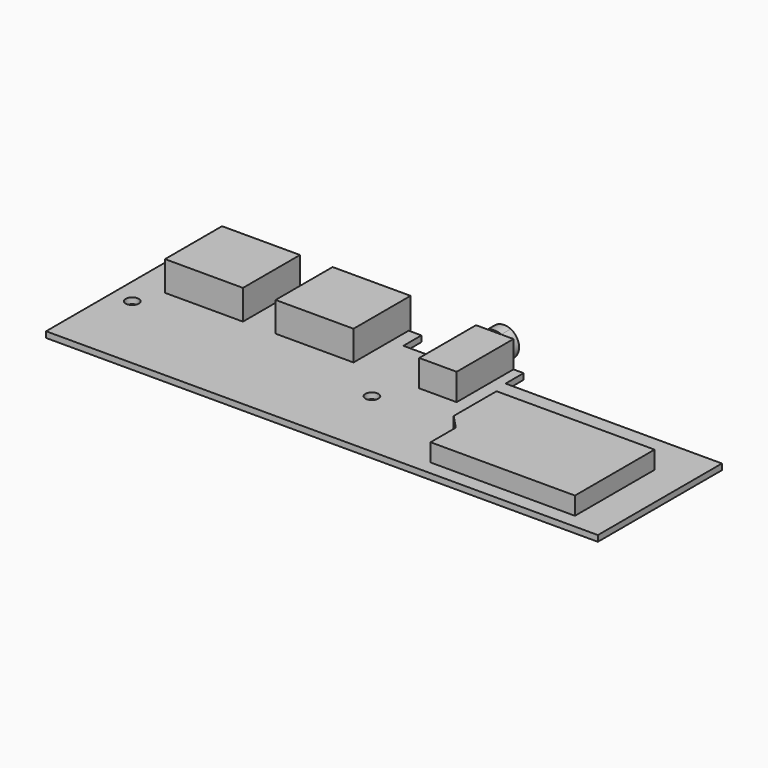
from build123d import *

# Parameters (mm, degrees)
F0_R      = 1.1
F1_DEPTH  = 1
F2_W      = 6.3
F2_H      = 11.95
F3_DEPTH  = 4.5
F4_DEPTH  = 3
F5_R      = 1.75
F6_DEPTH  = 2
F7_W      = 13.12
F7_H      = 5
F7_H_2    = 1
F8_DEPTH  = 12
F9_W      = 13.12
F9_H      = 5
F9_H_2    = 1
F10_DEPTH = 12


with BuildPart() as f1:
    # F0 (on Top) → F1 (new body)
    with BuildSketch(Plane.XY):
        Polygon((92.88, 0), (92.88, 26.1), (56.46, 26.1), (56.46, 29.9), (46.66, 29.9), (46.66, 26.1), (39.26, 26.1), (39.26, 29.9), (37.11, 29.9), (37.11, 18.3), (23.99, 18.3), (23.99, 28.9), (18.5, 28.9), (18.5, 18.3), (5.38, 18.3), (5.38, 29.9), (0.95, 29.9), (0.95, 26.6), (0, 26.6), (0, 0), align=None)
        with Locations((3.5, 13.75)):
            Circle(F0_R, mode=Mode.SUBTRACT)
        with Locations((45, 12.31)):
            Circle(F0_R, mode=Mode.SUBTRACT)
    extrude(amount=F1_DEPTH)

    # F2 (on face) → F3 (join)
    with BuildSketch(Plane.XY.offset(1)):
        with Locations((51.6, 23.925000114)):
            Rectangle(F2_W, F2_H)
    extrude(amount=F3_DEPTH)

    # F2 (on face) → F4 (join)
    with BuildSketch(Plane.XY.offset(1)):
        Polygon((87.1, 2.400000114), (87.1, 19.150000114), (60.5, 19.150000114), (60.5, 10.150000114), (62.8, 7.700000114), (62.8, 2.400000114), align=None)
    extrude(amount=F4_DEPTH)

    # F5 (on face) → F6 (join)
    with BuildSketch(Plane(origin=(0, 29.9, 0), x_dir=(-1, 0, 0), z_dir=(0, 1, 0))):
        with BuildLine():
            ThreePointArc((-50.5102752641, 1), (-49.4817091985, 1.9222786135), (-49.1, 3.25))
            ThreePointArc((-49.1, 3.25), (-49.4817091985, 4.5777213865), (-50.5102752641, 5.5))
            Line((-50.5102752641, 5.5), (-52.6897247359, 5.5))
            ThreePointArc((-52.6897247359, 5.5), (-54.1, 3.25), (-52.6897247359, 1))
            Line((-52.6897247359, 1), (-50.5102752641, 1))
        make_face()
        with Locations((-51.6, 3.25)):
            Circle(F5_R, mode=Mode.SUBTRACT)
        with BuildLine():
            Line((-52.6897247359, 5.5), (-50.5102752641, 5.5))
            ThreePointArc((-50.5102752641, 5.5), (-51.6, 5.75), (-52.6897247359, 5.5))
        make_face()
        with BuildLine():
            ThreePointArc((-52.6897247359, 1), (-51.6, 0.75), (-50.5102752641, 1))
            Line((-50.5102752641, 1), (-52.6897247359, 1))
        make_face()
    extrude(amount=F6_DEPTH)

    # F7 (on face) → F8 (join)
    with BuildSketch(Plane(origin=(0, 18.3, 0), x_dir=(-1, 0, 0), z_dir=(0, 1, 0))):
        with Locations((-11.94, 3.5)):
            Rectangle(F7_W, F7_H)
        with Locations((-11.94, 0.5)):
            Rectangle(F7_W, F7_H_2)
    extrude(amount=F8_DEPTH)

    # F9 (on face) → F10 (join)
    with BuildSketch(Plane(origin=(0, 18.3, 0), x_dir=(-1, 0, 0), z_dir=(0, 1, 0))):
        with Locations((-30.55, 3.5)):
            Rectangle(F9_W, F9_H)
        with Locations((-30.55, 0.5)):
            Rectangle(F9_W, F9_H_2)
    extrude(amount=F10_DEPTH)


solid = f1.part
